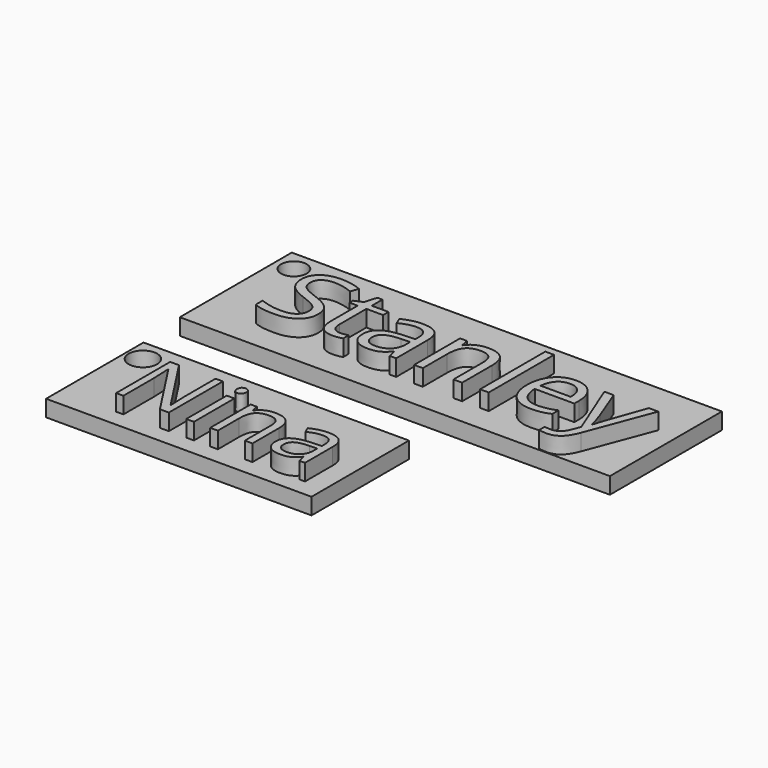
from build123d import *

# Parameters (mm, degrees)
F0_W          = 112.1814362705
F0_H          = 41.6195485741
F1_DEPTH      = 5
F2_R          = 3.8969930673
F3_DEPTH      = 25
F5_DEPTH      = 18.75
F4_TEXT_SIZE  = 32.6980603859
F6_DEPTH      = 5
F7_DEPTH      = 1
F8_W          = 128.5426057875
F8_H          = 35.0784738548
F9_DEPTH      = 5
F10_R         = 4.3410435478
F11_DEPTH     = 25
F12_DEPTH     = 2
F13_TEXT_SIZE = 28.7742871377
F14_DEPTH     = 5
F15_DEPTH     = 47.75


# Not quite as in the source:
# - Text() gives the source's letters only with a copy of the font that has no kerning and outlines rounded to 1/6400 em; it was checked with that copy


with BuildPart() as f1:
    # F0 (on Top) → F1 (new body)
    with BuildSketch(Plane.XY):
        with Locations((-2.9899086803, 31.9322412834)):
            Rectangle(F0_W, F0_H)
    extrude(amount=F1_DEPTH)

    # F2 (on face) → F3 (cut)
    with BuildSketch(Plane.XY.offset(5)):
        with Locations((-53.4417070448, 46.4966371655)):
            Circle(F2_R)
    extrude(amount=-F3_DEPTH, mode=Mode.SUBTRACT)

    # F5 (add): a face of the model
    f5_faces = [f1.faces().sort_by_distance(p)[0] for p in [
        (53.1008094549, 31.9322412834, 2.5),
    ]]
    extrude(f5_faces, amount=F5_DEPTH)

    # F4 (on face) → F6 (join)
    with BuildSketch(Plane.XY.offset(5)):
        with Locations((-44.7309426963, 18.2455163449)):
            Text('Stanley', F4_TEXT_SIZE, font='Open Sans', text_align=(TextAlign.LEFT, TextAlign.BOTTOM))
    extrude(amount=F6_DEPTH)

    # F7 (add): a face of the model
    f7_faces = [f1.faces().sort_by_distance(p)[0] for p in [
        (6.3850913197, 11.1224669963, 2.5),
    ]]
    extrude(f7_faces, amount=F7_DEPTH)


with BuildPart() as f9:
    # F8 (on Top) → F9 (new body)
    with BuildSketch(Plane.XY):
        with Locations((6.5919291228, -24.9551569577)):
            Rectangle(F8_W, F8_H)
    extrude(amount=F9_DEPTH)

    # F10 (on face) → F11 (cut)
    with BuildSketch(Plane.XY.offset(5)):
        with Locations((-52.5000020862, -12.1244397014)):
            Circle(F10_R)
    extrude(amount=-F11_DEPTH, mode=Mode.SUBTRACT)

    # F12 (add): a face of the model
    f12_faces = [f9.faces().sort_by_distance(p)[0] for p in [
        (6.5919291228, -7.4159200303, 2.5),
    ]]
    extrude(f12_faces, amount=F12_DEPTH)

    # F13 (on face) → F14 (join)
    with BuildSketch(Plane.XY.offset(5)):
        with Locations((-43.318387121, -37.3150222003)):
            Text('Nina', F13_TEXT_SIZE, font='Open Sans', text_align=(TextAlign.LEFT, TextAlign.BOTTOM))
    extrude(amount=F14_DEPTH)

    # F15 (cut): a face of the model
    f15_faces = [f9.faces().sort_by_distance(p)[0] for p in [
        (70.8632320166, -23.9551569577, 2.5),
    ]]
    extrude(f15_faces, amount=-F15_DEPTH, mode=Mode.SUBTRACT)


solid = Compound([f1.part, f9.part])
